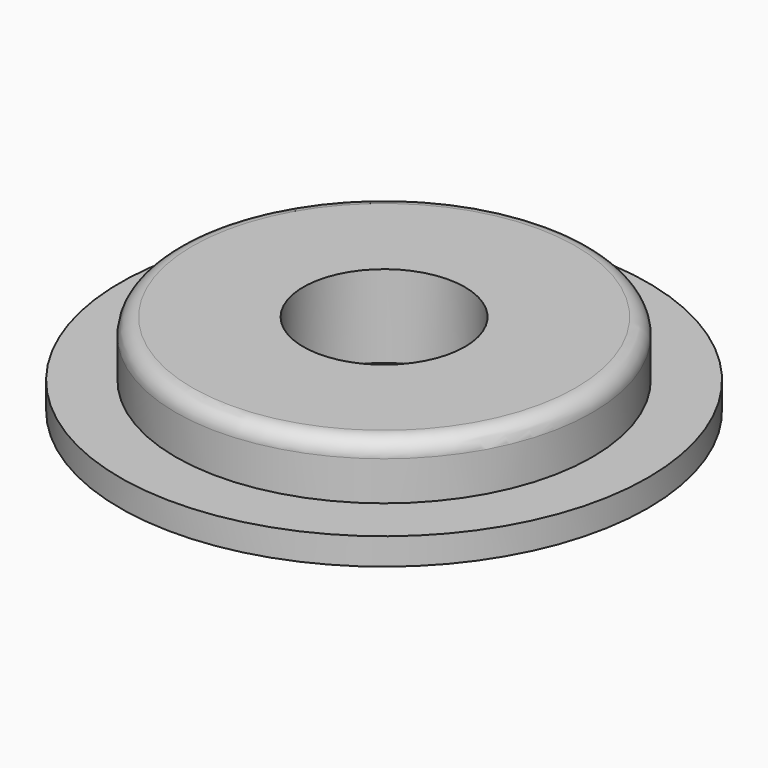
from build123d import *

# Parameters (mm, degrees)
F0_R     = 25.25
F0_R_2   = 12
F0_R_3   = 9.8
F1_DEPTH = 10
F0_R_4   = 32
F2_DEPTH = 3.25
F3_R     = 2


# Not quite as in the source:
# - a feature names something its author has since deleted; it is built from what else it names


with BuildPart() as f1:
    # F0 (on Top) → F1 (new body)
    with BuildSketch(Plane.XY):
        Circle(F0_R)
        Circle(F0_R_2, mode=Mode.SUBTRACT)
        Circle(F0_R_2)
        Circle(F0_R_3, mode=Mode.SUBTRACT)
    extrude(amount=F1_DEPTH)

    # F0 (on Top) → F2 (join)
    with BuildSketch(Plane.XY):
        Circle(F0_R_4)
        Circle(F0_R, mode=Mode.SUBTRACT)
    extrude(amount=F2_DEPTH)

    # F3
    f3_edges = [f1.edges().sort_by_distance(p)[0] for p in [
        (-25.25, 0, 10),
    ]]
    fillet(f3_edges, radius=F3_R)


solid = f1.part
